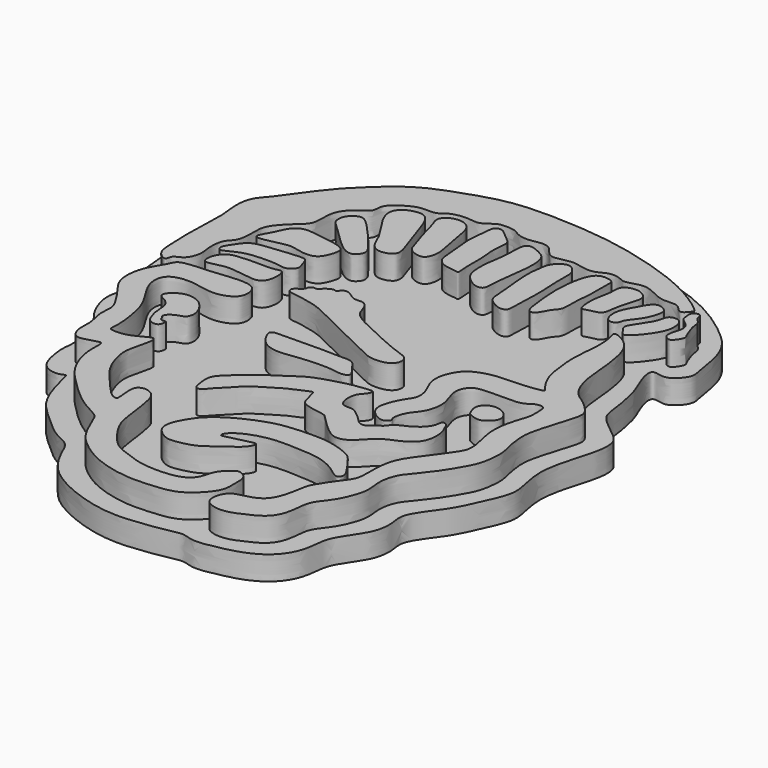
from build123d import *

# Parameters (mm, degrees)
F1_DEPTH     = 6.35
F3_DEPTH     = 6.35
F4_TEXT_SIZE = 8.8194444444
F5_DEPTH     = 3.175


# Not quite as in the source:
# - Text() gives the source's letters only with a copy of the font that has no kerning and outlines rounded to 1/6400 em; it was checked with that copy


with BuildPart() as f1:
    # F0 (on Top) → F1 (new body)
    with BuildSketch(Plane.XY):
        with BuildLine():
            add(Edge.make_bspline(
                [(57.3420971632, 19.5309109986), (58.6007502694, 17.8350979225), (63.1631906982, 14.7837725119), (65.7192379605, 11.7266263405), (65.2852353432, 6.5171671063), (63.3124977677, 0.5374782672), (61.7401040248, -6.2464160099), (62.0117362585, -11.2223538792), (63.3456826845, -16.3676346598), (63.2617116481, -20.0199297136), (60.3628025667, -26.6907168304), (57.5562496822, -32.4900621007), (54.1990561112, -36.694448129), (51.2332879467, -41.4674748525), (52.3532145245, -45.0370244781), (51.9247130212, -49.0842918835), (50.542552227, -52.2674079701), (46.1511647205, -58.284220045), (45.8206379188, -61.8232250464), (45.1815153517, -66.8554312845), (42.1928131847, -71.533264546), (36.9190061974, -74.8304506441), (30.1154298909, -76.3967815792), (24.5682467984, -77.3020438311), (21.5958733999, -75.8875942309), (19.169030203, -76.4484698519), (15.3832968822, -77.1799004378), (10.7803103798, -77.8196987402), (1.4372473986, -78.6986431695), (-11.5386004578, -74.3001147734), (-18.3270708536, -69.0656107595), (-21.3897181133, -63.0094824689), (-22.8951534736, -59.1783924003), (-27.6108341497, -57.7311616171), (-33.844883634, -51.8684019497), (-39.8715576725, -46.4828272222), (-42.0281559513, -35.4994488765), (-42.3651483631, -35.4090104114), (-44.3295795813, -36.4314480811), (-47.7985799514, -35.4675949418), (-49.636180417, -32.5249478057), (-50.6387988722, -26.3222545771), (-49.5982826341, -22.797147053), (-51.9104284224, -17.3618339214), (-50.7365911944, -15.3368894224), (-55.417422314, -10.2213755207), (-57.1525107853, -5.9577477562), (-58.1266139176, -1.2377946547), (-55.1929679224, 4.7922227911), (-58.9088402877, 7.5970461167), (-59.7646110245, 15.4670058788), (-60.3184686644, 22.0867653284), (-58.4617364493, 34.4086905126), (-62.065535147, 40.9166718965), (-53.6052029027, 51.6099161176), (-48.7662150174, 57.4763435719), (-42.736348953, 64.6190596252), (-33.7234931566, 70.9898685332), (-24.6838984976, 75.6529656089), (-12.4244284146, 79.005119082), (2.1196359962, 80.1707845401), (18.4021235012, 78.3573963952), (39.3158809141, 73.1840819106), (51.0394492301, 65.1034937377), (57.7083292271, 58.6270218611), (58.9505798802, 49.0454253791), (60.0034364774, 45.2023387777), (56.8316595987, 41.7279054633), (54.4939986432, 41.307479364), (51.1157418137, 42.517563137), (52.0299388674, 37.5336845076), (54.8950895547, 32.0916521126), (56.0495576012, 23.818191622), (56.3660280486, 20.8459919844), (57.3420971632, 19.5309109986)],
                knots=[0, 0, 0, 0, 0.0153737105, 0.0263934228, 0.03863439, 0.0530173302, 0.0677878357, 0.0804324458, 0.0931050771, 0.1037819905, 0.1187860968, 0.1332435296, 0.1464129053, 0.1592672907, 0.1698562757, 0.1808219412, 0.1915637969, 0.206621935, 0.2173371489, 0.2296965349, 0.2427593985, 0.2566243799, 0.2716505769, 0.2848599345, 0.294578999, 0.30320025, 0.3140584686, 0.3261074005, 0.3432425015, 0.3640732496, 0.3805187042, 0.3948666639, 0.4057373289, 0.4176617821, 0.4338199984, 0.4509338519, 0.4685814442, 0.4706946746, 0.4784820423, 0.4888285012, 0.4991414892, 0.5129295098, 0.5240600627, 0.5370434732, 0.5449119164, 0.5589943301, 0.5714264865, 0.5836105166, 0.5971643865, 0.6081930292, 0.6234465075, 0.6386061206, 0.6579918991, 0.6725962307, 0.6922791077, 0.7083501106, 0.7252465887, 0.7438778399, 0.7618093415, 0.7816926147, 0.8030182202, 0.8260013671, 0.8521321383, 0.8732019966, 0.8900348636, 0.907068579, 0.9180221242, 0.9293181588, 0.9381247609, 0.9468424262, 0.9573308866, 0.9720114511, 0.9880778874, 1, 1, 1, 1], degree=3))
        make_face()
    extrude(amount=-F1_DEPTH)

    # F2 (on Top) → F3 (join)
    with BuildSketch(Plane.XY):
        with BuildLine():
            add(Edge.make_bspline(
                [(-27.8626866639, 37.7302952111), (-26.5948488448, 36.5245322897), (-24.9553026523, 35.0970190076), (-22.2896591809, 34.2008549465), (-20.6245032961, 36.1097855669), (-20.5625130615, 37.8343057887), (-23.1887841131, 41.2522964732), (-28.0898662924, 46.8527501901), (-29.9652758139, 48.4000448395), (-31.557219679, 49.138615945), (-34.5784235934, 47.0206882949), (-34.3393753913, 43.769310011), (-32.8753101088, 42.6914630589), (-29.5239765084, 39.3102462631), (-27.8626866639, 37.7302952111)],
                knots=[0, 0, 0, 0, 0.0955897208, 0.1674561834, 0.2358612461, 0.2928333978, 0.3899286566, 0.5203144924, 0.5927632596, 0.6494141727, 0.7337437652, 0.8118641407, 0.874745626, 1, 1, 1, 1], degree=3))
        make_face()
        with BuildLine():
            add(Edge.make_bspline(
                [(-23.0002496392, 44.4088205695), (-22.4209720095, 43.3219543573), (-21.919777866, 41.6565041752), (-20.1906789893, 39.2932102196), (-17.7436662316, 39.0492593034), (-15.3614268378, 39.9935228425), (-14.8527149343, 42.0883352347), (-16.7984721121, 47.0165364519), (-18.6855093935, 52.8659555397), (-20.0794978279, 56.5771009518), (-22.3716361977, 58.2688353189), (-26.7355835964, 57.0946632228), (-28.1958320217, 54.6151732048), (-27.7811957868, 52.1553112819), (-26.2542213259, 49.2590546017), (-23.7968846488, 45.903502275), (-23.0002496392, 44.4088205695)],
                knots=[0, 0, 0, 0, 0.068995189, 0.1324683654, 0.1921125308, 0.2517087692, 0.3037871831, 0.3933064251, 0.4933426271, 0.5698258813, 0.6314997006, 0.7111345672, 0.7745838826, 0.8332765921, 0.9051163376, 1, 1, 1, 1], degree=3))
        make_face()
        with BuildLine():
            add(Edge.make_bspline(
                [(-17.5519771874, 55.3053691983), (-17.8497891968, 56.1608562303), (-18.659880099, 57.763409061), (-17.3914596919, 59.7240926638), (-14.3822686309, 60.7923578106), (-11.3324947074, 59.5850470367), (-10.2308052017, 56.5006711445), (-9.4561587357, 50.8871216768), (-8.2267672678, 46.0537872841), (-9.364247451, 42.853825453), (-11.3130379641, 42.4794456604), (-14.204762177, 43.720070693), (-14.8013970836, 46.2125902148), (-16.8209434976, 51.9937803348), (-17.2060337086, 54.3116209595), (-17.5519771874, 55.3053691983)],
                knots=[0, 0, 0, 0, 0.0682756406, 0.1281706627, 0.2023391042, 0.274944474, 0.3493628437, 0.4519712719, 0.5487827964, 0.6211263871, 0.6766250433, 0.7477658232, 0.8154707814, 0.9206898585, 1, 1, 1, 1], degree=3))
        make_face()
        with BuildLine():
            add(Edge.make_bspline(
                [(-7.3584350757, 54.4851981103), (-7.3587699473, 55.9397973329), (-6.8454384435, 60.0851270457), (-6.7450837326, 62.4066516813), (-4.6523965352, 62.7978586199), (-3.0973048694, 61.2310500613), (-1.3355256252, 59.8422184682), (0.113312732, 58.6022839439), (-0.8197853249, 54.6658969318), (0.0029405113, 50.2243253883), (-0.3431190506, 45.191370053), (0.1793763552, 41.8064641333), (-0.7436619625, 42.1728713744), (-4.2116951194, 42.3444964568), (-6.3697651643, 44.0742120263), (-6.7813838835, 46.8316245123), (-7.0328276748, 52.3709270984), (-7.3582225434, 53.5620101111), (-7.3584350757, 54.4851981103)],
                knots=[0, 0, 0, 0, 0.0882259293, 0.1419860519, 0.1880015183, 0.2421182561, 0.2980027918, 0.3451568684, 0.4156138894, 0.4956788903, 0.5819227787, 0.6425830924, 0.6694115441, 0.7380186103, 0.7970686187, 0.8585708595, 0.9440058005, 1, 1, 1, 1], degree=3))
        make_face()
        with BuildLine():
            add(Edge.make_bspline(
                [(2.1906888578, 49.0955077112), (2.353857072, 50.5912377548), (2.9362751386, 52.9969946904), (2.8755876114, 57.2793648258), (3.1566641175, 59.8901106714), (4.5694244219, 60.7947106081), (7.3146917425, 59.5944112815), (9.3806420283, 58.4124645772), (10.2707567007, 55.1634503359), (9.7161050593, 48.9493665343), (8.7045758081, 42.8744805375), (8.9446598935, 39.5547889419), (6.4911072422, 39.1549240878), (3.472725969, 41.2970163063), (1.9623033376, 43.774826967), (2.0063130508, 47.40537195), (2.1906888578, 49.0955077112)],
                knots=[0, 0, 0, 0, 0.0787909455, 0.1594474558, 0.2204353933, 0.2646490314, 0.3302855041, 0.3895217702, 0.4570707293, 0.5556615718, 0.6549725237, 0.7193389488, 0.7715321231, 0.8447507992, 0.9109682959, 1, 1, 1, 1], degree=3))
        make_face()
        with BuildLine():
            add(Edge.make_bspline(
                [(12.3842312023, 42.6513142884), (12.1774034805, 44.8486192684), (11.5536737171, 49.7091642142), (12.082309728, 54.2676860932), (12.6585786438, 57.0354101887), (15.3495263385, 59.0889212288), (17.2398528639, 58.4660076201), (18.6506454375, 56.6025695836), (18.6633414544, 54.5656430319), (18.5972920332, 51.0054986147), (18.8587693007, 47.6484649864), (18.9513588167, 43.9089531264), (18.6598112199, 40.2355330574), (18.6864900207, 36.8067179675), (18.5734410686, 35.1736029717), (17.3583299911, 34.6777517133), (15.8491833136, 34.9021313285), (13.0461906612, 36.5100214324), (12.6704361685, 38.656587402), (12.5409227815, 40.9866477521), (12.3842312023, 42.6513142884)],
                knots=[0, 0, 0, 0, 0.0878149403, 0.1580169156, 0.2121328472, 0.2687057505, 0.3120577239, 0.3599445024, 0.4063846288, 0.4678650678, 0.5288704152, 0.5918730957, 0.6558980323, 0.7168683892, 0.7561672692, 0.789737075, 0.8304458414, 0.8873015588, 0.9334718695, 1, 1, 1, 1], degree=3))
        make_face()
        with BuildLine():
            add(Edge.make_bspline(
                [(25.6241187453, 40.7180562615), (25.00543232, 39.8018272344), (24.1446313225, 37.4483584667), (21.9664376315, 37.422989676), (21.3633819149, 41.0853954143), (20.6642614752, 47.7804812558), (21.1396619917, 54.089484371), (22.5263276197, 58.3590456597), (24.6866992029, 59.5210848238), (27.9759037213, 58.9032682586), (27.4367008657, 56.6456616141), (27.9049760458, 52.2074707906), (27.052780661, 47.1021270299), (27.4575480021, 42.3906537528), (26.1282046681, 41.4645703852), (25.6241187453, 40.7180562615)],
                knots=[0, 0, 0, 0, 0.0759278154, 0.123211472, 0.1952590685, 0.3033984844, 0.4078584546, 0.4906472126, 0.5517706017, 0.6181373372, 0.6722480612, 0.7581627865, 0.8538395164, 0.9381364431, 1, 1, 1, 1], degree=3))
        make_face()
        with BuildLine():
            add(Edge.make_bspline(
                [(29.7835562378, 51.4388531446), (29.5915963548, 50.3737727087), (29.4387317394, 48.3701509329), (29.8183768351, 44.6952519844), (31.8647305344, 45.7855699798), (35.0621676137, 45.9322579488), (35.2662859939, 49.164931646), (36.3174070734, 53.6822492656), (37.6642769215, 57.0873427958), (35.1711733213, 58.8769329546), (33.1274498233, 59.0359417816), (30.225075275, 58.1577591538), (30.5763104123, 54.6462247637), (29.9767390414, 52.5107188982), (29.7835562378, 51.4388531446)],
                knots=[0, 0, 0, 0, 0.0899669105, 0.172656483, 0.2359536398, 0.318483099, 0.3993570217, 0.5085506143, 0.5974016153, 0.6743254067, 0.7459555049, 0.8231315411, 0.9094599365, 1, 1, 1, 1], degree=3))
        make_face()
        with BuildLine():
            add(Edge.make_bspline(
                [(36.7550030351, 48.2753403485), (36.9268750846, 49.8870610005), (38.5070657483, 52.4516828407), (40.170707418, 55.8578139176), (42.0433216293, 56.7064604191), (44.5495926434, 55.3362143757), (44.3241118821, 53.2371558044), (43.102101597, 49.5912729971), (40.1552939447, 46.6404303184), (40.1991272831, 44.6627557933), (37.2634977028, 43.9813128807), (36.600117932, 46.8229138485), (36.7550030351, 48.2753403485)],
                knots=[0, 0, 0, 0, 0.1278427366, 0.2408872934, 0.3193568129, 0.4101916784, 0.4899306805, 0.6069052843, 0.7262909203, 0.8023067057, 0.8847925797, 1, 1, 1, 1], degree=3))
        make_face()
        with BuildLine():
            add(Edge.make_bspline(
                [(43.0820323527, 42.8856499493), (42.7157046726, 43.4066277959), (41.7581914689, 44.3752677937), (43.5971913354, 46.9844619237), (46.2657111339, 51.0307989419), (46.2645934492, 53.8956189709), (49.7379931684, 54.295537263), (50.6447987831, 50.9632563189), (50.1193777314, 48.1279017945), (48.1494202558, 44.9651634791), (45.9097484705, 42.2665708179), (44.0749988931, 41.1308785555), (43.4510081331, 42.3609060712), (43.0820323527, 42.8856499493)],
                knots=[0, 0, 0, 0, 0.0713966776, 0.1636646272, 0.287327238, 0.3735463024, 0.4590655017, 0.5526642353, 0.6466466021, 0.7530435006, 0.8583801356, 0.9280872119, 1, 1, 1, 1], degree=3))
        make_face()
        with BuildLine():
            add(Edge.make_bspline(
                [(-41.1611609161, 32.2234369814), (-40.5519271652, 33.4168545421), (-40.0015619234, 35.417168875), (-37.1747693836, 37.5901308126), (-33.4505391945, 36.8147733201), (-28.3049723137, 36.342232117), (-25.2701406439, 35.119033626), (-25.1758393482, 33.0987630329), (-26.4915657484, 29.421296716), (-28.9487008909, 28.495012581), (-31.8725571087, 28.8683530064), (-34.636961988, 29.7848011332), (-39.0184620636, 28.4723278806), (-42.4290684817, 27.9500035559), (-43.2268265642, 28.927677017), (-41.7996811763, 30.9726505791), (-41.1611609161, 32.2234369814)],
                knots=[0, 0, 0, 0, 0.076057159, 0.1471740943, 0.2257891166, 0.3207730164, 0.3898918958, 0.4434511388, 0.5221204683, 0.585617529, 0.65431826, 0.72337164, 0.8121379886, 0.8857018257, 0.9202866931, 1, 1, 1, 1], degree=3))
        make_face()
        with BuildLine():
            add(Edge.make_bspline(
                [(-44.0317578614, 22.8500645608), (-44.6443513802, 21.9591465128), (-45.8433259786, 20.4535345633), (-45.1618797566, 18.4680073513), (-42.3898412074, 20.1015765937), (-39.0724884288, 21.4625548747), (-31.6523263231, 21.6274323242), (-29.2422522076, 20.6355105016), (-26.5954077218, 22.5035905265), (-27.7313137284, 24.7863057327), (-28.0707386361, 26.8957872357), (-30.6608671635, 26.9729615582), (-36.7215864457, 26.2854021103), (-42.2474684751, 25.7896310625), (-43.4092918057, 23.7553406144), (-44.0317578614, 22.8500645608)],
                knots=[0, 0, 0, 0, 0.0748627648, 0.1232893437, 0.1912145418, 0.27764898, 0.3933858181, 0.4627402591, 0.5297390169, 0.5945978871, 0.653051801, 0.715229309, 0.8243928941, 0.9239307494, 1, 1, 1, 1], degree=3))
        make_face()
        with BuildLine():
            add(Edge.make_bspline(
                [(-44.2075058818, 16.1129534245), (-43.903110406, 16.8734358583), (-42.8743386488, 18.4533149628), (-39.729952857, 19.1288907657), (-34.5913270644, 19.2200994203), (-30.8599171977, 19.0074986796), (-28.5959910739, 20.0443854752), (-27.9461090257, 16.8517895226), (-28.8292356464, 13.6043342547), (-31.1507490463, 12.8116226249), (-35.1721134729, 13.51113646), (-38.8480207255, 14.0029420639), (-41.6842051142, 13.1843142685), (-44.1904207656, 12.6947825465), (-44.7048138326, 14.1940719617), (-44.4828282319, 15.4251054518), (-44.2075058818, 16.1129534245)],
                knots=[0, 0, 0, 0, 0.0670669726, 0.1416576574, 0.2396257595, 0.3235165835, 0.3802036129, 0.4484355242, 0.5252513091, 0.5870627155, 0.673039078, 0.7557558672, 0.8301817315, 0.8930252675, 0.9393386631, 1, 1, 1, 1], degree=3))
        make_face()
        with BuildLine():
            add(Edge.make_bspline(
                [(-40.7510772347, 10.1960124448), (-38.9137599882, 10.311767208), (-36.5829233108, 10.7106018865), (-32.4684434858, 10.9936562163), (-28.3057247016, 10.3714491848), (-27.7984145907, 5.5610260688), (-30.667832239, 3.4942610034), (-34.4037095803, 2.795758626), (-38.0284757865, 3.6121294078), (-41.9338611212, 4.3049630514), (-46.5527353202, 3.1326737422), (-47.2994800941, -0.735664015), (-45.8766621849, -4.3543968169), (-43.0786878914, -8.4607142873), (-41.4176754846, -12.1360293375), (-40.140197161, -20.0827073392), (-40.7390034082, -22.8530312262), (-39.7321205679, -23.2389644403), (-36.8343935528, -23.2990666704), (-33.8845886768, -22.0014528446), (-31.938254735, -20.8278284353), (-30.6196202823, -20.4994331508), (-30.1199832798, -22.3146127791), (-32.2939083687, -28.2669716006), (-31.3171416977, -32.6657772506), (-29.5971353669, -37.2490045536), (-25.6707790496, -41.6680573642), (-21.7371997364, -46.316939762), (-20.0920032649, -46.5819052805), (-19.7382535068, -45.9776680139), (-20.2614954214, -42.3927038722), (-20.0478335439, -40.1649939602), (-17.9750077682, -39.1864193425), (-15.1540856859, -40.4208065228), (-14.101051314, -43.5516695873), (-13.2501232442, -49.9139022002), (-12.5888453933, -55.2376658428), (-9.1086525063, -60.0960582941), (-6.3535164779, -63.3167219535), (-1.6882776561, -64.920088672), (2.1732999564, -66.3921065441), (8.2620599062, -66.6896425796), (13.0144953795, -65.9241331975), (15.8541849705, -63.5600234112), (16.3065425043, -59.3948795534), (18.9093058011, -57.2257091349), (20.2511672175, -56.017743249), (23.181296124, -57.3913702408), (23.1176739141, -60.8088559395), (23.3645424349, -65.0809576857), (19.5238339545, -69.4515466508), (15.7105048092, -71.9855225218), (10.6732133189, -72.58997487), (3.9775078834, -72.9857923556), (-1.9678437414, -71.7534853914), (-7.3089801248, -69.9213242087), (-13.1986975346, -65.6730508119), (-15.8067368708, -61.9407742846), (-17.7706527955, -56.8397459351), (-18.8800195859, -54.9577552231), (-23.6151497586, -52.8807224992), (-28.2975130481, -48.9334737965), (-32.8934207275, -44.4871184419), (-36.2309642397, -40.1882677663), (-38.1071008025, -34.1077844503), (-37.7020297342, -30.1442982302), (-37.9853108683, -28.8568664524), (-39.1841395467, -29.1344334421), (-41.3806102842, -29.7504055007), (-44.1838606391, -30.5581001276), (-45.9616839644, -27.2123344662), (-45.1995155419, -23.253216561), (-46.8495126424, -18.7422733722), (-45.909799231, -15.4231778412), (-47.5765177921, -12.1772947531), (-50.1694062024, -8.4148622761), (-53.2031425584, -4.6381382101), (-52.7704800693, 2.3221084739), (-49.1858380654, 7.2545059195), (-48.5518991237, 10.0409130904), (-43.1311744938, 10.0460614251), (-40.7510772347, 10.1960124448)],
                knots=[0, 0, 0, 0, 0.0134485435, 0.0264032426, 0.0387068811, 0.0512386913, 0.0627453773, 0.0751329549, 0.0874713233, 0.100453096, 0.1136903698, 0.1253888902, 0.1380919208, 0.1521760985, 0.1655438033, 0.1838858401, 0.1938671954, 0.19938508, 0.2101861186, 0.2220152069, 0.2317945708, 0.2382439014, 0.245687772, 0.2617596743, 0.2755724503, 0.2894547134, 0.3055662953, 0.3213507402, 0.3284284844, 0.3328546266, 0.345042518, 0.3546082206, 0.3633959754, 0.3739332964, 0.3853577184, 0.4016569408, 0.4167822764, 0.4322094495, 0.4454479939, 0.4593648876, 0.4726034334, 0.4884371958, 0.5025171432, 0.5142487135, 0.5271038223, 0.5386881962, 0.5468321794, 0.5570471709, 0.5684952747, 0.5816619769, 0.5967915854, 0.6104569429, 0.6247730926, 0.641492484, 0.6572814322, 0.6726735046, 0.6897225485, 0.7038046103, 0.7184807523, 0.7278083469, 0.7419230699, 0.7581990618, 0.7744130768, 0.7894645007, 0.8057033928, 0.8184636457, 0.8246620899, 0.830903468, 0.840943685, 0.8511780069, 0.862378107, 0.8754228422, 0.8892995874, 0.9008639713, 0.912767273, 0.9265778069, 0.9404990842, 0.9570855084, 0.9727928195, 0.9825784896, 1, 1, 1, 1], degree=3))
        make_face()
        with BuildLine():
            add(Edge.make_bspline(
                [(-54.4596351683, 14.706951566), (-54.393625757, 13.0712346964), (-54.3274185117, 10.4715056086), (-51.8895360111, 8.6715423096), (-51.014273571, 8.9108294259), (-50.9798267765, 10.4720449067), (-49.5212887603, 11.0709856048), (-47.8096276876, 12.0511060789), (-46.732466354, 15.4296938963), (-47.3695054506, 17.8060660055), (-47.3450207438, 20.8642113993), (-46.5472365361, 23.1755066555), (-44.4803697506, 24.6991557199), (-44.3439073298, 29.7321309171), (-44.4425348033, 33.0879508403), (-40.8394448064, 37.0474891658), (-38.2847560067, 39.0787546428), (-37.0009711173, 41.0088373367), (-37.4169360425, 45.953748076), (-35.7031447595, 49.0593562158), (-33.5210224828, 50.9728815504), (-30.7253661594, 52.3160848987), (-31.2664042837, 55.3918979536), (-28.6362108796, 57.6372227733), (-25.4972423888, 59.5938384946), (-22.6445675163, 59.8098353562), (-19.8559161723, 59.7036151544), (-18.733805984, 61.2243795351), (-15.0782749354, 62.3712896568), (-12.1447595774, 61.9696264693), (-10.1939503645, 61.8007377818), (-7.8356886263, 63.6697466996), (-6.5080043127, 64.3880584992), (-2.531226527, 64.3054727855), (-1.3334622419, 63.0793388101), (1.7027561886, 62.1992442969), (4.8034211846, 63.0885917234), (7.880575258, 62.9224021076), (9.4632353913, 60.0291566499), (11.4873440767, 59.3468056382), (15.2290519703, 60.4909381681), (17.1503274952, 60.2150786194), (19.6632354389, 59.5650369089), (22.3175323912, 59.6865653488), (24.67003703, 61.3697174783), (27.6276096302, 61.1344687716), (29.3232675998, 59.9023779637), (32.1356234292, 60.9941030066), (34.9111329512, 61.4517080434), (38.3891850445, 59.7026239807), (40.9762462488, 58.5577291233), (44.9097914116, 59.2755506859), (46.1429743326, 57.275339835), (47.5668342569, 56.618327256), (48.8610634172, 58.3631041536), (49.64085628, 59.1962207931), (42.9527463883, 63.9263177019), (35.3417940717, 67.4802549684), (24.7156090951, 70.8333316211), (13.6588702022, 73.0978651593), (0.0214389242, 74.0420946236), (-11.633732324, 73.629502473), (-21.3606082569, 70.4070735979), (-31.4586251249, 66.7785308732), (-39.2584772362, 59.5763375238), (-44.5639402157, 54.2781797493), (-51.0248165612, 44.5226003711), (-54.6560677383, 41.060799916), (-55.0019219234, 35.8117660252), (-54.0907803884, 31.7981976356), (-54.8397669304, 22.103993183), (-54.5469566361, 16.8707823756), (-54.4596351683, 14.706951566)],
                knots=[0, 0, 0, 0, 0.0153082888, 0.0270819566, 0.0328646989, 0.0412849728, 0.050127762, 0.0603779114, 0.0737675054, 0.0855285815, 0.0983107396, 0.1095673049, 0.1208862805, 0.1369559042, 0.1506501293, 0.1673272193, 0.1807082536, 0.191481429, 0.2076106662, 0.2214163716, 0.2340178951, 0.2461861529, 0.2580221827, 0.2713222026, 0.2855425934, 0.2981338477, 0.3098949217, 0.3196007268, 0.3337987704, 0.3465846109, 0.3567184858, 0.3690101278, 0.3785192863, 0.3926195459, 0.4023449285, 0.4149336051, 0.42837842, 0.4407358224, 0.4534223565, 0.4638330121, 0.4781452732, 0.4885898719, 0.5002921738, 0.5121880733, 0.5245779696, 0.536853001, 0.5471174127, 0.5593966052, 0.5718174013, 0.5860591492, 0.5987506988, 0.612737057, 0.6233955878, 0.6315736305, 0.6418921568, 0.648015063, 0.6674894778, 0.6901353907, 0.7144576628, 0.739495668, 0.7668503536, 0.7920565898, 0.8155639481, 0.8397859592, 0.8634031088, 0.8842088057, 0.909213575, 0.9257342067, 0.9416048564, 0.9568266186, 0.9797492172, 1, 1, 1, 1], degree=3))
        make_face()
        with BuildLine():
            add(Edge.make_bspline(
                [(51.7477020621, 48.9783398807), (51.9972879859, 49.8810840975), (52.6078471378, 51.5144707736), (51.4702261511, 53.5544891786), (49.4128509502, 54.5064369627), (49.3672709096, 56.4418394347), (49.113284529, 57.77928164), (50.8573202971, 58.7599893727), (51.5094653495, 58.0012363211), (51.5369343181, 56.7137507852), (53.2881460105, 55.4914328846), (53.2898344556, 53.4100896224), (53.9476944105, 51.5991606257), (54.7359485289, 49.2887950965), (55.5126813744, 48.3869989136), (53.9597701408, 46.0421089528), (53.1163486559, 45.5318777485), (51.1949514931, 46.4733166644), (51.5093310259, 48.1161595497), (51.7477020621, 48.9783398807)],
                knots=[0, 0, 0, 0, 0.0724266123, 0.1372199727, 0.2018999356, 0.2612110549, 0.3115956774, 0.3679818138, 0.406642022, 0.4556092633, 0.5179846272, 0.5803002453, 0.6441341657, 0.7132887504, 0.7590385198, 0.8302255289, 0.8736265341, 0.9308278032, 1, 1, 1, 1], degree=3))
        make_face()
        with BuildLine():
            add(Edge.make_bspline(
                [(43.3501154184, 20.4309597611), (43.0764725087, 22.2407283905), (42.4946409225, 26.8007524479), (43.3631516012, 32.9199168492), (43.3215400137, 38.0000037183), (42.2965219057, 40.5834170266), (43.1914956973, 40.8800166676), (46.4296881717, 39.3160207988), (48.7347901345, 36.2669320871), (49.7191314916, 31.7996634431), (50.3630009263, 27.2570911593), (50.6127736978, 21.3328284112), (52.7132076836, 14.9055503712), (56.685125614, 12.7707288445), (59.1226103721, 10.3439623061), (60.5182382244, 8.2938090439), (59.2973304556, 4.1464951556), (57.3416312372, -2.2056202112), (56.2161913441, -6.831473543), (57.0278561957, -12.2918392702), (58.224110808, -16.0678563004), (57.4007425773, -21.7936257366), (56.0141954272, -24.8330569238), (52.2406722501, -31.1046187375), (48.7284720907, -35.0662466544), (46.8706249483, -37.6036788837), (45.8560586565, -41.8060029606), (46.784441533, -45.8449985784), (45.7904100441, -49.7528078677), (43.8698626487, -54.0845446891), (40.6210898632, -57.6299844931), (40.2175892655, -60.714561036), (39.8303649342, -64.8402082638), (37.8894488028, -68.4671286899), (33.2727338882, -70.8123323664), (29.0536817223, -72.4796441053), (25.3726824662, -71.9492947349), (23.5553037061, -70.5135688743), (23.3589917701, -67.6750146854), (24.9327989382, -64.9844412205), (26.9816682313, -64.4996954625), (29.575179257, -63.8833320934), (32.4292926009, -62.6699253076), (34.4733491912, -59.2057809583), (35.2352142712, -54.1733748025), (35.7337399501, -51.7511319522), (39.0545281049, -46.783517627), (41.9239268729, -43.4628161204), (41.5159587295, -38.628903422), (42.0205765726, -33.1058545826), (44.2299247011, -29.2686648493), (47.2570352932, -25.3607279455), (49.9464013674, -21.5154114244), (51.8541864435, -18.6554219204), (50.9143388282, -14.0227812599), (50.0763389345, -10.9000006485), (49.9321024316, -6.6375695502), (51.2619244936, -1.6619173644), (52.263891634, 0.8366617313), (52.1404542863, 4.1361511576), (51.9627109197, 5.9669380524), (49.3605585995, 5.8602286793), (47.6845291042, 4.1028414244), (43.5902916146, 3.873656618), (37.5861966836, 4.0449419845), (34.5852429175, 3.4984219431), (32.9157447598, 1.0548619271), (33.0910648523, -1.8376625853), (35.068334875, -6.0425607026), (33.7442492506, -11.431198511), (30.9788014142, -13.7674930909), (30.0143621806, -17.7797698886), (31.0063059668, -18.4189047547), (29.7063174819, -20.2266243933), (26.780592946, -19.0753214598), (24.6845459827, -16.7849889964), (24.9787661254, -13.5007104353), (26.8148939802, -9.5341753876), (28.7281847954, -7.2809451934), (28.2280665607, -3.7089903198), (26.354663372, -0.7401042155), (25.9459166563, 3.085355149), (27.9741551431, 7.5030545673), (30.8102539146, 9.3905399634), (35.0044959085, 10.6222885851), (40.7333064939, 10.628756297), (45.3003493506, 11.012231513), (47.3152896612, 11.500246125), (47.094560912, 12.1253582917), (45.9860822087, 13.2491953123), (43.9776949277, 16.7211335706), (43.5658115335, 19.0044288746), (43.3501154184, 20.4309597611)],
                knots=[0, 0, 0, 0, 0.0144970142, 0.0291253682, 0.0423615193, 0.051042932, 0.0551455571, 0.0657188152, 0.0771756262, 0.0893437693, 0.1017322369, 0.1159516192, 0.1306491445, 0.1426946121, 0.1532765055, 0.1618006498, 0.1734473434, 0.1885163938, 0.2012848161, 0.2145153848, 0.226248967, 0.2396785548, 0.2505057517, 0.2660601286, 0.2794805262, 0.2895657991, 0.301291581, 0.3129858609, 0.3244197826, 0.3370980397, 0.3495439089, 0.3595837737, 0.3712071714, 0.3826821185, 0.3956900771, 0.4081077999, 0.4189034954, 0.4271910114, 0.436556243, 0.4463876298, 0.4545338131, 0.4639387015, 0.4738782639, 0.4853609568, 0.4982172847, 0.5074749678, 0.5213686463, 0.5334142756, 0.545799413, 0.5593532623, 0.5714286773, 0.5843236789, 0.5968516366, 0.6073159247, 0.6194681493, 0.629989914, 0.6418915353, 0.6549314358, 0.6645751805, 0.6749829754, 0.6820114416, 0.6902403481, 0.6990164318, 0.7105702065, 0.7249326987, 0.7347836856, 0.7440172487, 0.7535919905, 0.7659648645, 0.7790649822, 0.7903416174, 0.8012851559, 0.8064887167, 0.81362753, 0.8233093848, 0.8332228821, 0.8433795389, 0.8554608413, 0.8652132905, 0.8756446478, 0.8864639379, 0.8976125015, 0.9100349265, 0.9204940468, 0.9324028786, 0.9464467695, 0.9591392183, 0.9664674521, 0.9700269305, 0.9771277182, 0.9885728827, 1, 1, 1, 1], degree=3))
        make_face()
        with BuildLine():
            add(Edge.make_bspline(
                [(-7.9300757498, 9.0172849596), (-9.8292378314, 9.9872647023), (-13.4151444252, 11.9442720829), (-19.5895814194, 13.0161896033), (-22.248378701, 13.220419714), (-22.4542352626, 14.8839850294), (-20.6519361204, 15.7238846482), (-19.9620551774, 16.6940404323), (-20.153881988, 17.3584261198), (-19.0048198063, 18.0261014199), (-17.7971079773, 17.565359251), (-17.2828480254, 18.8935623821), (-16.6834067308, 19.114150854), (-15.3226233808, 19.9871989573), (-14.3054037518, 19.3039292755), (-13.9216931676, 20.643644998), (-12.4431880169, 21.018023245), (-10.8440967631, 20.0036253974), (-9.3288101694, 18.9128122464), (-7.5770964643, 19.3299551655), (-5.9255651502, 18.6971941465), (-5.1019766391, 16.7027339466), (-4.5141399713, 14.6814032593), (-2.500877696, 12.8973626305), (2.2454308463, 10.725852905), (7.5301819919, 8.2180696289), (12.2724685123, 6.2183834324), (15.2622524583, 5.4146170644), (16.00687957, 3.6502964949), (15.3804049719, 1.5484901466), (12.7705437182, 0.4206904861), (9.0015765794, 0.5362732622), (6.0531107647, 2.3769769929), (1.0901436485, 4.578871975), (-2.5296365723, 6.36774772), (-6.0871670257, 8.0760361071), (-7.9300757498, 9.0172849596)],
                knots=[0, 0, 0, 0, 0.0481937077, 0.0961672905, 0.1249477574, 0.1448636289, 0.1710842859, 0.1911521791, 0.2052788054, 0.225440353, 0.2455684655, 0.2657824813, 0.281524814, 0.304904048, 0.3227441833, 0.3421221208, 0.3640181763, 0.3900973774, 0.4157319742, 0.4404814739, 0.4645716411, 0.4919666649, 0.519308707, 0.5495573188, 0.5930827986, 0.6403176044, 0.6840101983, 0.7163184249, 0.7405493274, 0.7669917353, 0.7980988258, 0.8343597906, 0.8702146914, 0.9141993103, 0.9532337944, 1, 1, 1, 1], degree=3))
        make_face()
        with BuildLine():
            add(Edge.make_bspline(
                [(-35.3384241462, -12.2506394982), (-35.4755204255, -12.0017043974), (-35.9279658301, -11.6665808908), (-35.1117694211, -10.2470721741), (-33.0332173852, -9.3217069375), (-31.3310994887, -8.9917991704), (-30.7766994168, -6.4273073254), (-32.0435712339, -3.7730222272), (-33.9480744039, -1.6511250863), (-37.2415572292, -0.6883204091), (-39.7616563325, -1.6783453754), (-41.6376700894, -3.2569389559), (-41.8337197523, -4.8764452865), (-40.0275121234, -5.4927509501), (-38.3056633992, -6.9991029957), (-38.0830127765, -9.2705864018), (-37.9520882373, -11.5139973678), (-37.2663577484, -13.2758196633), (-36.791037003, -14.8094106598), (-35.2615061367, -15.5068532396), (-33.6692975261, -15.353737901), (-33.4383239872, -13.791144405), (-33.3439740785, -13.0429145001), (-34.990596472, -13.5450224995), (-35.1663965303, -12.5630018184), (-35.3384241462, -12.2506394982)],
                knots=[0, 0, 0, 0, 0.0276409271, 0.0652396603, 0.1152068207, 0.1561442779, 0.2048072212, 0.2606286689, 0.3156399609, 0.3741643606, 0.4276483551, 0.478012805, 0.5141289952, 0.556562391, 0.6051944089, 0.6537715735, 0.7030435098, 0.7480427497, 0.7883010761, 0.8293031067, 0.8672891667, 0.9064569366, 0.9291528416, 0.9653163251, 1, 1, 1, 1], degree=3))
        make_face()
        with BuildLine():
            add(Edge.make_bspline(
                [(-2.6107039303, -52.9527589679), (-3.3036671535, -52.4278381632), (-4.5969957008, -51.1129996681), (-4.515668735, -47.6556474443), (-1.937804719, -43.6741372681), (-0.7190498421, -42.0269374418), (3.1080763556, -38.7975063632), (9.4033446867, -35.8272215434), (14.649999852, -34.2890391249), (21.7023904463, -33.9277207131), (27.1983242038, -34.1169450807), (32.5759607807, -36.0451382644), (34.3639082232, -37.4165338463), (37.1515242885, -41.3780265405), (38.830098644, -43.8967807272), (38.0566662122, -45.8519804331), (35.9573677055, -44.7620596297), (34.1751288338, -43.0572828348), (29.485348862, -40.9451661397), (23.6824992675, -40.7909953449), (17.4693019264, -40.36559707), (11.2472176902, -41.9401503557), (8.1691410072, -43.91787936), (7.1573216897, -45.2772749058), (7.275377724, -46.2519272785), (8.9393663365, -45.6583370508), (12.1769251826, -44.9303378932), (14.922426975, -44.2722762064), (15.729780129, -44.5334539676), (14.8417903803, -47.0065368976), (10.9300044998, -49.394312644), (6.8660119058, -52.9787324913), (2.8510265558, -53.8459378044), (-0.2474013283, -54.4037709578), (-1.9023760708, -53.4893185102), (-2.6107039303, -52.9527589679)],
                knots=[0, 0, 0, 0, 0.0258137024, 0.0551435771, 0.0900412168, 0.113552924, 0.1490797539, 0.1923125829, 0.2307550071, 0.273426905, 0.3126493881, 0.3502797981, 0.3749377979, 0.4105884899, 0.4389314606, 0.4579080986, 0.4798626888, 0.5060522171, 0.542148872, 0.5816026086, 0.6225756198, 0.6637568462, 0.6945657321, 0.7147690995, 0.727289519, 0.7462654827, 0.7775494865, 0.8046850708, 0.8160704381, 0.8391386577, 0.8746290023, 0.9126906818, 0.945400034, 0.9736139467, 1, 1, 1, 1], degree=3))
        make_face()
        with BuildLine():
            add(Edge.make_bspline(
                [(41.467115283, -5.8363941498), (41.2993881644, -5.476307405), (40.2676688387, -3.4873323954), (41.4317839933, -1.0303649183), (43.9906850433, -0.2605619916), (46.3179869477, -0.9949815999), (47.8421586722, -2.5027831719), (48.2488475301, -4.5007799449), (46.7560266265, -6.2366354828), (44.5134037709, -7.6884287815), (41.5859397201, -6.1546638874), (41.5312831467, -5.9741536091), (41.467115283, -5.8363941498)],
                knots=[0, 0, 0, 0, 0.1072920221, 0.2172310075, 0.3263814315, 0.4335450445, 0.5337409786, 0.627111812, 0.7289034879, 0.8412751035, 0.9589529713, 1, 1, 1, 1], degree=3))
        make_face()
        with BuildLine():
            add(Edge.make_bspline(
                [(-1.9286716124, -8.7267933413), (-3.7482197526, -8.9433991078), (-6.1902150392, -9.4615113356), (-10.6510601295, -8.7882620498), (-12.9321415879, -5.979617464), (-14.1161573728, -3.3166745155), (-11.8013124025, -2.717940358), (-7.4977766193, -3.0850142416), (-0.6564573298, -2.6844082469), (4.0465710571, -2.9804732827), (7.6979137231, -2.746262527), (8.9061948966, -4.287087467), (10.8154220659, -6.7073663284), (11.5251879368, -8.3477632139), (9.3519998993, -9.0833783892), (6.2561774344, -8.1008241913), (0.5288593786, -8.4342397275), (-1.9286716124, -8.7267933413)],
                knots=[0, 0, 0, 0, 0.0761294885, 0.1485812566, 0.2170649341, 0.2710012196, 0.3168697072, 0.3924870856, 0.4872532291, 0.5670716032, 0.6317428678, 0.6799657799, 0.7439340973, 0.7857747335, 0.8314677422, 0.8971774513, 1, 1, 1, 1], degree=3))
        make_face()
        with BuildLine():
            add(Edge.make_bspline(
                [(-4.0939841419, -27.4157300591), (-4.7724674096, -28.1205031058), (-7.6677268647, -30.7535273216), (-8.3687856962, -32.2547190327), (-10.3584406196, -32.9760495894), (-10.8072549968, -29.9562727989), (-11.0420255598, -27.5088678695), (-10.1269806777, -25.662819698), (-7.8965083647, -23.6199129747), (-5.0861008982, -21.0427954389), (-1.6554633656, -18.4721377494), (1.3574698994, -16.7178884503), (3.9300479182, -14.7271554336), (6.9546067584, -13.3234945018), (10.8636538409, -12.2328106647), (14.1216144839, -11.2637672324), (18.6504491072, -10.7392939628), (19.8996458382, -10.7704693018), (19.4491269327, -12.4997111129), (17.745474301, -13.7919007719), (17.3355370825, -16.4343982332), (17.6767172257, -18.4288715271), (18.7900423695, -19.8439468714), (21.3317787483, -19.4326525185), (22.9203104809, -20.6379514141), (24.5612037263, -21.9261228979), (26.2382085357, -23.9347551705), (27.9447288521, -24.0662651803), (29.4563954982, -22.6612800119), (31.5603696291, -21.3460801571), (32.0708219026, -19.9244171747), (33.7104256085, -19.2365149768), (35.3689996932, -18.4902550227), (37.5740766356, -17.06142639), (38.6742431626, -15.7234075462), (39.3866584258, -14.3232618192), (39.336461633, -12.61863676), (40.7796636915, -12.6906809837), (41.4307038575, -14.2248035591), (42.4757404038, -16.2901022968), (42.5062869535, -19.1854549213), (41.9587704688, -21.9281690065), (39.2517541675, -24.3533619225), (36.1655850877, -25.5126694474), (33.817641224, -26.7426454539), (31.6844804256, -28.8648668748), (29.8570574361, -31.0568139683), (26.6452362842, -32.3103223002), (23.831615117, -30.7241177201), (21.040912973, -28.1509626534), (18.9931334246, -25.9930753909), (18.2428260449, -25.3026078462), (15.0435180208, -24.9146933512), (11.4966731861, -24.0897669864), (11.0586589719, -21.6246107748), (10.4796263419, -19.5828060314), (10.1814831878, -18.6740207146), (8.5794744166, -19.4424193594), (5.4029101847, -20.6212482775), (2.0056761138, -22.7657314533), (-1.4561761095, -24.7889660299), (-3.5644144105, -26.7478629163), (-3.7983653891, -27.1086567103), (-4.0939841419, -27.4157300591)],
                knots=[0, 0, 0, 0, 0.0230007878, 0.0374380405, 0.0496749547, 0.0663861116, 0.0833802481, 0.0979035085, 0.1160291664, 0.1369009427, 0.1588017426, 0.178537198, 0.1973499003, 0.2166401672, 0.2376120251, 0.2579146045, 0.2803747468, 0.2900091892, 0.3021509717, 0.3176738284, 0.3345103359, 0.3494813166, 0.362531549, 0.378626095, 0.3931764267, 0.408666115, 0.4254511819, 0.4380844213, 0.4530857421, 0.4696216058, 0.4820906794, 0.4955262051, 0.5100996972, 0.527099628, 0.5409742252, 0.5542685959, 0.5667992897, 0.5770069461, 0.5901387911, 0.606286094, 0.6240731217, 0.6414478537, 0.6611008701, 0.6803109755, 0.6974039773, 0.715501029, 0.7334606454, 0.7519955594, 0.770301032, 0.7914061711, 0.8091955332, 0.8194059279, 0.8381519946, 0.8577393708, 0.8735895859, 0.8891587365, 0.8977232679, 0.9101748855, 0.9299299536, 0.9513570292, 0.9729713765, 0.989978435, 1, 1, 1, 1], degree=3))
        make_face()
    extrude(amount=F3_DEPTH)

    # F4 (on face) → F5 (cut)
    with BuildSketch(Plane(origin=(0, 0, -6.35), x_dir=(1, 0, 0), z_dir=(0, 0, -1))):
        with Locations(Location((2.8918569923, 69.822024497), (0, 0, -140))):
            Text('Riley Frisell', F4_TEXT_SIZE, font='Arimo', font_style=FontStyle.BOLD, text_align=(TextAlign.LEFT, TextAlign.BOTTOM))
    extrude(amount=-F5_DEPTH, mode=Mode.SUBTRACT)


solid = f1.part
